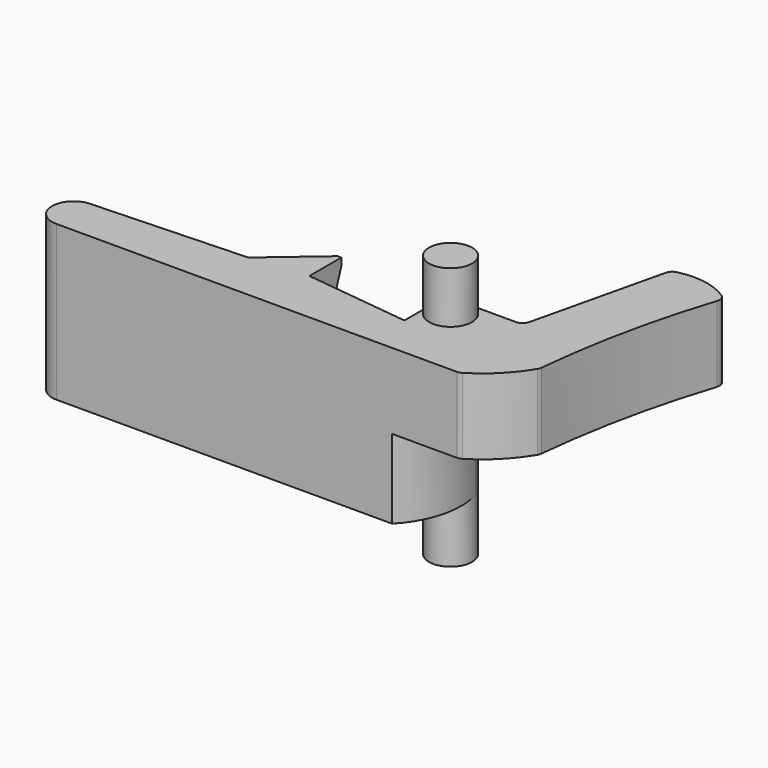
from build123d import *

# Parameters (mm, degrees)
F1_DEPTH = 5.715
F2_R     = 1.5875
F3_DEPTH = 4.1656
F4_R     = 1.5875
F5_DEPTH = 3.81
F7_DEPTH = 5.842


with BuildPart() as f1:
    # F0 (on Top) → F1 (new body, symmetric)
    with BuildSketch(Plane.XY):
        with BuildLine():
            Line((3.5549216614, 1.5875), (0, 1.5875))
            ThreePointArc((0, 1.5875), (-1.1225320151, 1.1225320151), (-1.5875, 0))
            Line((-1.5875, 0), (-1.5875, -2.2225))
            Line((-1.5875, -2.2225), (-9.3345, -1.3589))
            Line((-9.3345, -1.3589), (-9.3345, 1.5875))
            Line((-9.3345, 1.5875), (-9.608742781, 1.5875))
            Line((-9.608742781, 1.5875), (-13.5255, -1.7653))
            Line((-13.5255, -1.7653), (-24.8539, -2.2225))
            ThreePointArc((-24.8539, -2.2225), (-26.3770597496, -3.8407239016), (-24.7898826087, -5.3962086948))
            Line((-24.7898826087, -5.3962086948), (4.7834118114, -5.3962086948))
            ThreePointArc((4.7834118114, -5.3962086948), (4.9527721319, -5.3729059822), (5.1095456268, -5.3047296971))
            ThreePointArc((5.1095456268, -5.3047296971), (6.8320364553, -3.9473788403), (8.1809379528, -2.2182632419))
            ThreePointArc((8.1809379528, -2.2182632419), (8.238795955, -2.0926103635), (8.2676969204, -1.9573294393))
            ThreePointArc((8.2676969204, -1.9573294393), (9.2733035869, 4.537554361), (10.9688257926, 10.8873547355))
            ThreePointArc((10.9688257926, 10.8873547355), (10.9628913183, 11.2928057385), (10.7101033421, 11.6098608961))
            ThreePointArc((10.7101033421, 11.6098608961), (8.8799829062, 12.3144977387), (6.9200560471, 12.2471137853))
            ThreePointArc((6.9200560471, 12.2471137853), (6.6220302078, 12.0799126553), (6.4559206195, 11.7812770521))
            Line((6.4559206195, 11.7812770521), (4.1652633995, 2.0706188245))
            ThreePointArc((4.1652633995, 2.0706188245), (3.9441262464, 1.7228965355), (3.5549216614, 1.5875))
        make_face()
    extrude(amount=F1_DEPTH, both=True)

    # F2 (on face) → F3 (join)
    with BuildSketch(Plane(origin=(0, 0, -5.715), x_dir=(1, 0, 0), z_dir=(0, 0, -1))):
        Circle(F2_R)
    extrude(amount=F3_DEPTH)

    # F4 (on face) → F5 (join)
    with BuildSketch(Plane.XY.offset(5.715)):
        Circle(F4_R)
    extrude(amount=F5_DEPTH)

    # F6 (on face) → F7 (cut)
    with BuildSketch(Plane(origin=(0, 0, -5.715), x_dir=(1, 0, 0), z_dir=(0, 0, -1))):
        with BuildLine():
            Line((9.2012649402, 17.4278523773), (0, 5.3962086948))
            ThreePointArc((0, 5.3962086948), (1.5278567181, 2.7004632752), (1.5367644299, -0.3981348225))
            ThreePointArc((1.5367644299, -0.3981348225), (0.9716267852, -1.255427274), (0, -1.5875))
            Line((0, -1.5875), (-3.6485670134, -20.050900057))
            Line((-3.6485670134, -20.050900057), (23.1213513762, -22.8752493858))
            Line((23.1213513762, -22.8752493858), (9.2012649402, 17.4278523773))
        make_face()
    extrude(amount=-F7_DEPTH, mode=Mode.SUBTRACT)

    # F8 (on Top) → F9 (revolve, cut)
    with BuildSketch(Plane.XY):
        Polygon((-9.3345, -2.3811933066), (-1.5875, -3.2447933066), (-1.5875, 2.2244379615), (-13.4883278617, 2.3323959991), (-13.5255, -1.7653), (-9.608742781, 0.5715), (-9.3345, 0.5715), align=None)
    revolve(axis=Axis((0.2309344709, 14.1097, 0), (1, 0, 0)), mode=Mode.SUBTRACT)


solid = f1.part
